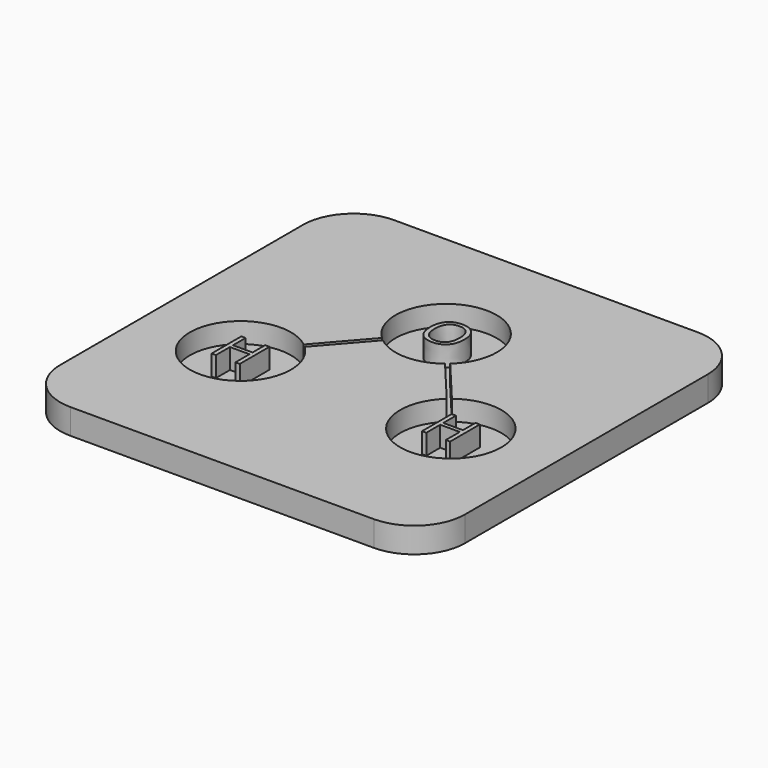
from build123d import *

# Parameters (mm, degrees)
F1_DEPTH     = 0.635
F3_DEPTH     = 3.175
F4_TEXT_SIZE = 6.5220733328
F5_DEPTH     = 2.54
F6_DEPTH     = 2.54


# Not quite as in the source:
# - a feature names something its author has since deleted; it is built from what else it names
# - Text() gives the source's letters only with a copy of the font that has no kerning and outlines rounded to 1/6400 em; it was checked with that copy


with BuildPart() as f1:
    # F0 (on Top) → F1 (new body)
    with BuildSketch(Plane.XY):
        with BuildLine():
            Line((19.05, 25.4), (-19.05, 25.4))
            ThreePointArc((-19.05, 25.4), (-23.5401280605, 23.5401280605), (-25.4, 19.05))
            Line((-25.4, 19.05), (-25.4, -19.05))
            ThreePointArc((-25.4, -19.05), (-23.5401280605, -23.5401280605), (-19.05, -25.4))
            Line((-19.05, -25.4), (19.05, -25.4))
            ThreePointArc((19.05, -25.4), (23.5401280605, -23.5401280605), (25.4, -19.05))
            Line((25.4, -19.05), (25.4, 19.05))
            ThreePointArc((25.4, 19.05), (23.5401280605, 23.5401280605), (19.05, 25.4))
        make_face()
    extrude(amount=F1_DEPTH)

    # F2 (on face) → F3 (cut)
    with BuildSketch(Plane.XY.offset(0.635)):
        with BuildLine():
            Line((-3.9805307961, 4.7927855023), (-3.9772833376, 4.7966902621))
            ThreePointArc((-3.9772833376, 4.7966902621), (-0.0615476987, 3.3971114994), (3.880581911, 4.7205239248))
            Line((3.880581911, 4.7205239248), (8.6706442988, -0.9956174603))
            ThreePointArc((8.6706442988, -0.9956174603), (17.0191174539, -10.5626679018), (9.0600077686, -0.6693352383))
            Line((9.0600077686, -0.6693352383), (4.2699453808, 5.0468061467))
            ThreePointArc((4.2699453808, 5.0468061467), (0.0612197004, 16.096518102), (-4.3597719873, 5.1300082358))
            Line((-4.3597719873, 5.1300082358), (-4.3635025598, 5.1265468366))
            Line((-4.3635025598, 5.1265468366), (-9.4776118512, -0.7415968159))
            Line((-9.4776118512, -0.7415968159), (-9.4810188999, -0.7453733537))
            ThreePointArc((-9.4810188999, -0.7453733537), (-17.6300821383, -10.4828388424), (-9.0980643982, -1.0791087798))
            Line((-9.0980643982, -1.0791087798), (-9.0946400875, -1.0753581501))
            Line((-9.0946400875, -1.0753581501), (-3.9805307961, 4.7927855023))
        make_face()
    extrude(amount=F3_DEPTH, mode=Mode.SUBTRACT)

    # F2 (on face) → F6 (join)
    with BuildSketch(Plane.XY.offset(0.635)):
        with BuildLine():
            ThreePointArc((19.05, -25.4), (23.5401280605, -23.5401280605), (25.4, -19.05))
            Line((25.4, -19.05), (25.4, 19.05))
            ThreePointArc((25.4, 19.05), (23.5401280605, 23.5401280605), (19.05, 25.4))
            Line((19.05, 25.4), (-19.05, 25.4))
            ThreePointArc((-19.05, 25.4), (-23.5401280605, 23.5401280605), (-25.4, 19.05))
            Line((-25.4, 19.05), (-25.4, -19.05))
            ThreePointArc((-25.4, -19.05), (-23.5401280605, -23.5401280605), (-19.05, -25.4))
            Line((-19.05, -25.4), (19.05, -25.4))
        make_face()
        with BuildLine():
            ThreePointArc((3.880581911, 4.7205239248), (-0.0615476987, 3.3971114994), (-3.9772833376, 4.7966902621))
            Line((-3.9772833376, 4.7966902621), (-3.9805307961, 4.7927855023))
            Line((-3.9805307961, 4.7927855023), (-9.0946400875, -1.0753581501))
            Line((-9.0946400875, -1.0753581501), (-9.0980643982, -1.0791087798))
            ThreePointArc((-9.0980643982, -1.0791087798), (-17.6300821383, -10.4828388424), (-9.4810188999, -0.7453733537))
            Line((-9.4810188999, -0.7453733537), (-9.4776118512, -0.7415968159))
            Line((-9.4776118512, -0.7415968159), (-4.3635025598, 5.1265468366))
            Line((-4.3635025598, 5.1265468366), (-4.3597719873, 5.1300082358))
            ThreePointArc((-4.3597719873, 5.1300082358), (0.0612197004, 16.096518102), (4.2699453808, 5.0468061467))
            Line((4.2699453808, 5.0468061467), (9.0600077686, -0.6693352383))
            ThreePointArc((9.0600077686, -0.6693352383), (17.0191174539, -10.5626679018), (8.6706442988, -0.9956174603))
            Line((8.6706442988, -0.9956174603), (3.880581911, 4.7205239248))
        make_face(mode=Mode.SUBTRACT)
    extrude(amount=F6_DEPTH)


with BuildPart() as f5:
    # F4 (on face) → F5 (new body)
    with BuildSketch(Plane.XY.offset(0.635)):
        with Locations((-15.9716513008, -7.8769173285)):
            Text('H', F4_TEXT_SIZE, font='Open Sans', text_align=(TextAlign.LEFT, TextAlign.BOTTOM))
        with Locations((10.4259896796, -7.8769173285)):
            Text('H', F4_TEXT_SIZE, font='Open Sans', text_align=(TextAlign.LEFT, TextAlign.BOTTOM))
        with Locations((-2.5146, 7.5655204157)):
            Text('O', F4_TEXT_SIZE, font='Open Sans', text_align=(TextAlign.LEFT, TextAlign.BOTTOM))
    extrude(amount=F5_DEPTH)


solid = Compound([f1.part, f5.part])
